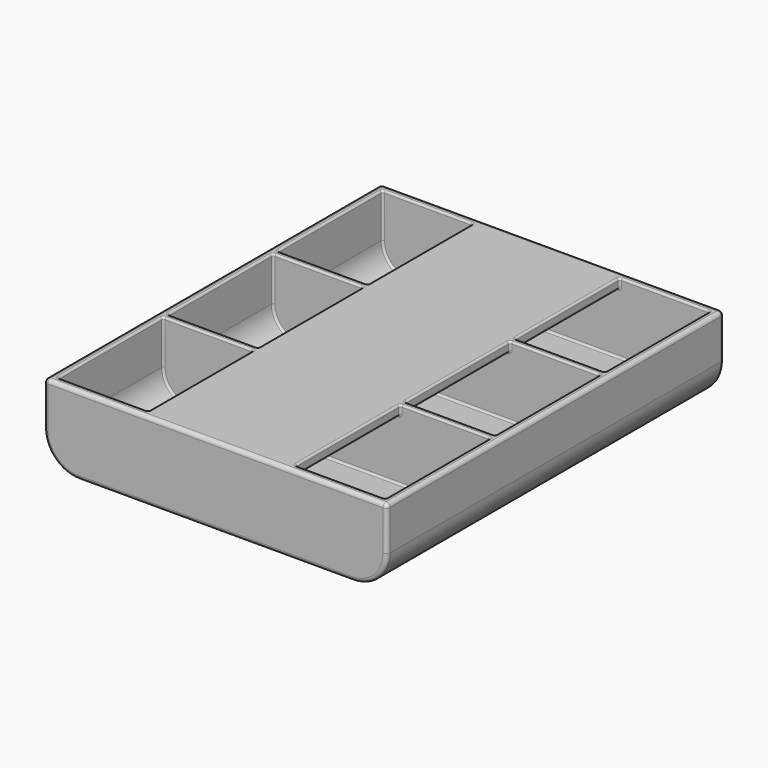
from build123d import *

# Parameters (mm, degrees)
F1_DEPTH  = 207
F3_DEPTH  = 4
F5_DEPTH  = 4
F9_DEPTH  = 3
F11_DEPTH = 3
F12_W     = 75
F12_H     = 5
F13_DEPTH = 207
F14_F1_R  = 1
F14_F2_R  = 1
F14_F3_R  = 1
F14_F4_R  = 1
F15_R     = 2


with BuildPart() as f1:
    # F0 (on Front) → F1 (new body)
    with BuildSketch(Plane.XZ):
        with BuildLine():
            Line((-87.0672343036, 3.9621459596), (-91.0672343036, 3.9621459596))
            Line((-91.0672343036, 3.9621459596), (-91.0672343036, -18.3878540309))
            ThreePointArc((-91.0672343036, -18.3878540309), (-85.8976689888, -30.8682887255), (-73.4172342941, -36.0378540404))
            Line((-73.4172342941, -36.0378540404), (66.2827657059, -36.0378540404))
            ThreePointArc((66.2827657059, -36.0378540404), (78.7632003877, -30.868288725), (83.9327656964, -18.3878540404))
            Line((83.9327656964, -18.3878540404), (83.9327656964, 3.9621459596))
            Line((83.9327656964, 3.9621459596), (79.9327656964, 3.9621459596))
            Line((79.9327656964, 3.9621459596), (79.9327656964, -18.3878540404))
            ThreePointArc((79.9327656964, -18.3878540404), (75.9347732629, -28.0398616002), (66.2827657059, -32.0378540404))
            Line((66.2827657059, -32.0378540404), (-73.4172342941, -32.0378540404))
            ThreePointArc((-73.4172342941, -32.0378540404), (-83.069241864, -28.0398616008), (-87.0672343036, -18.3878540309))
            Line((-87.0672343036, -18.3878540309), (-87.0672343036, 3.9621459596))
        make_face()
    extrude(amount=F1_DEPTH)

    # F2 (on face) → F3 (join)
    with BuildSketch(Plane.XZ.offset(207)):
        with BuildLine():
            Line((83.9327656964, 3.9621459596), (-91.0672343036, 3.9621459596))
            Line((-91.0672343036, 3.9621459596), (-91.0672343036, -18.3878540309))
            ThreePointArc((-91.0672343036, -18.3878540309), (-85.8976689888, -30.8682887255), (-73.4172342941, -36.0378540404))
            Line((-73.4172342941, -36.0378540404), (66.2827657059, -36.0378540404))
            ThreePointArc((66.2827657059, -36.0378540404), (78.7632003877, -30.868288725), (83.9327656964, -18.3878540404))
            Line((83.9327656964, -18.3878540404), (83.9327656964, 3.9621459596))
        make_face()
    extrude(amount=F3_DEPTH)

    # F4 (on face) → F5 (join)
    with BuildSketch(Plane(origin=(0, 0, 0), x_dir=(-1, 0, 0), z_dir=(0, 1, 0))):
        with BuildLine():
            Line((-83.9327656964, 3.9621459596), (-83.9327656964, -18.3878540404))
            ThreePointArc((-83.9327656964, -18.3878540404), (-78.7632003877, -30.868288725), (-66.2827657059, -36.0378540404))
            Line((-66.2827657059, -36.0378540404), (73.4172342941, -36.0378540404))
            ThreePointArc((73.4172342941, -36.0378540404), (85.8976689888, -30.8682887255), (91.0672343036, -18.3878540309))
            Line((91.0672343036, -18.3878540309), (91.0672343036, 3.9621459596))
            Line((91.0672343036, 3.9621459596), (-83.9327656964, 3.9621459596))
        make_face()
    extrude(amount=F5_DEPTH)

    # F8 (on offset) → F9 (join)
    with BuildSketch(Plane.XZ.offset(67)):
        with BuildLine():
            Line((-87.0672343036, 3.9621459596), (-87.0672343036, -18.3878540309))
            ThreePointArc((-87.0672343036, -18.3878540309), (-83.069241864, -28.0398616008), (-73.4172342941, -32.0378540404))
            Line((-73.4172342941, -32.0378540404), (66.2827656964, -32.0378540404))
            ThreePointArc((66.2827656964, -32.0378540404), (75.9347732596, -28.0398616036), (79.9327656964, -18.3878540404))
            Line((79.9327656964, -18.3878540404), (79.9327656964, 3.9621459596))
            Line((79.9327656964, 3.9621459596), (-87.0672343036, 3.9621459596))
        make_face()
    extrude(amount=F9_DEPTH)

    # F10 (on offset) → F11 (join)
    with BuildSketch(Plane.XZ.offset(137)):
        with BuildLine():
            Line((-87.0647428878, 3.9621459596), (-87.0647428878, -18.1270678269))
            ThreePointArc((-87.0647428878, -18.1270678269), (-83.1610074839, -27.9472151123), (-73.4172342941, -32.0378540404))
            Line((-73.4172342941, -32.0378540404), (66.2827656964, -32.0378540404))
            ThreePointArc((66.2827656964, -32.0378540404), (76.0641632523, -27.9087133427), (79.9277927893, -18.0194308688))
            Line((79.9277927893, -18.0194308688), (79.9277927893, 3.9621459596))
            Line((79.9277927893, 3.9621459596), (-87.0647428878, 3.9621459596))
        make_face()
    extrude(amount=F11_DEPTH)

    # F12 (on face) → F13 (join)
    with BuildSketch(Plane.XZ):
        with Locations((-3.5672343036, 1.4621459596)):
            Rectangle(F12_W, F12_H)
    extrude(amount=F13_DEPTH)

    # F14: fillet of radius 1 on 76 edges, made by hand

    # F14_f1
    f14_f1_edges = [f1.edges().sort_by_distance(p)[0] for p in [
        (-87.0672343036, 0, -7.2128540356),
        (79.9327656964, -70, -7.2128540404),
        (75.9347732596, -140, -28.0398616036),
        (-87.0672343036, -67, -7.2128540356),
        (-83.069241864, -137, -28.0398616008),
        (-87.0672343036, -207, -7.2128540356),
        (-83.069241864, 0, -28.0398616008),
        (-3.5672342941, 0, -32.0378540404),
        (75.9347732629, 0, -28.0398616002),
        (79.9327656964, 0, -7.2128540404),
        (79.9327656964, -67, -7.2128540404),
        (75.9347732596, -67, -28.0398616036),
        (-3.5672342989, -67, -32.0378540404),
        (-83.069241864, -67, -28.0398616008),
        (75.9347732596, -70, -28.0398616036),
        (-3.5672342989, -70, -32.0378540404),
        (-83.069241864, -70, -28.0398616008),
        (-87.0672343036, -70, -7.2128540356),
        (79.9327656964, -207, -7.2128540404),
        (75.9347732629, -207, -28.0398616002),
        (-3.5672342941, -207, -32.0378540404),
        (-83.069241864, -207, -28.0398616008),
        (75.9347732596, -137, -28.0398616036),
        (-3.5672342989, -137, -32.0378540404),
        (-3.5672342989, -140, -32.0378540404),
        (-83.069241864, -140, -28.0398616008),
    ]]
    fillet(f14_f1_edges, radius=F14_F1_R)

    # F14_f2
    f14_f2_edges = [f1.edges().sort_by_distance(p)[0] for p in [
        (33.9327656964, -173.5, -1.0378540404),
        (33.9327656964, -103.5, -1.0378540404),
        (-41.0672343036, -173.5, -1.0378540404),
        (-41.0672343036, -103.5, -1.0378540404),
        (-41.0672343036, -33.5, -1.0378540404),
        (33.9327656964, -33.5, -1.0378540404),
    ]]
    fillet(f14_f2_edges, radius=F14_F2_R)

    # F14_f3
    f14_f3_edges = [f1.edges().sort_by_distance(p)[0] for p in [
        (-41.0672343036, -70, 1.9621459596),
        (-41.0672343036, -140, 1.9621459596),
        (33.9327656964, -140, 1.9621459596),
        (33.9327656964, -207, 1.9621459596),
        (33.9327656964, -137, 1.9621459596),
        (33.9327656964, -67, 1.9621459596),
        (33.9327656964, 0, 1.9621459596),
        (-3.5672343036, 0, -1.0378540404),
        (-41.0672343036, 0, 1.9621459596),
        (-41.0672343036, -67, 1.9621459596),
        (-3.5672343036, -67, -1.0378540404),
        (-3.5672343036, -70, -1.0378540404),
        (33.9327656964, -70, 1.9621459596),
        (-41.0672343036, -207, 1.9621459596),
        (-3.5672343036, -207, -1.0378540404),
        (-41.0672343036, -137, 1.9621459596),
        (-3.5672343036, -137, -1.0378540404),
        (-3.5672343036, -140, -1.0378540404),
        (33.6398724776, -140, -0.7449608215),
        (-40.7743410848, -140, -0.7449608215),
        (33.6398724776, -137, -0.7449608215),
        (-40.7743410848, -137, -0.7449608215),
        (-40.7743410848, -207, -0.7449608215),
        (33.6398724776, -207, -0.7449608215),
        (33.6398724776, -70, -0.7449608215),
        (-40.7743410848, -70, -0.7449608215),
        (33.6398724776, -67, -0.7449608215),
        (-40.7743410848, -67, -0.7449608215),
        (-40.7743410848, 0, -0.7449608215),
        (33.6398724776, 0, -0.7449608215),
    ]]
    fillet(f14_f3_edges, radius=F14_F3_R)

    # F14_f4
    f14_f4_edges = [f1.edges().sort_by_distance(p)[0] for p in [
        (79.9327656964, -103.5, 3.9621459596),
        (79.9327656964, -173.5, 3.9621459596),
        (-87.0672343036, -173.5, 3.9621459596),
        (-87.0672343036, -103.5, 3.9621459596),
        (-87.0672343036, -33.5, 3.9621459596),
        (79.9327656964, -33.5, 3.9621459596),
        (79.6398724776, -0.2928932188, 3.9621459596),
        (79.6398724776, -66.7071067812, 3.9621459596),
        (-86.7743410848, -0.2928932188, 3.9621459596),
        (-86.7743410848, -66.7071067812, 3.9621459596),
        (-86.7743410848, -70.2928932188, 3.9621459596),
        (-86.7743410881, -136.7071067843, 3.9621459596),
        (-86.7743410881, -140.2928932157, 3.9621459596),
        (-86.7743410848, -206.7071067812, 3.9621459596),
        (79.6398724809, -140.2928932157, 3.9621459596),
        (79.6398724776, -206.7071067812, 3.9621459596),
        (79.6398724776, -70.2928932188, 3.9621459596),
        (79.6398724809, -136.7071067843, 3.9621459596),
    ]]
    fillet(f14_f4_edges, radius=F14_F4_R)

    # F15
    f15_edges = [f1.edges().sort_by_distance(p)[0] for p in [
        (83.932766, -211, -7.212854),
        (-3.567234, -211, 3.962146),
        (83.932766, -103.5, 3.962146),
        (-91.067234, -103.5, 3.962146),
        (83.932766, 4, -7.212854),
        (-3.567234, 4, 3.962146),
        (-91.067234, -211, -7.212854),
        (-85.897669, -211, -30.868289),
        (-3.567234, -211, -36.037854),
        (78.7632, -211, -30.868289),
        (-91.067234, 4, -7.212854),
        (78.7632, 4, -30.868289),
        (-3.567234, 4, -36.037854),
        (-85.897669, 4, -30.868289),
    ]]
    fillet(f15_edges, radius=F15_R)


solid = f1.part
